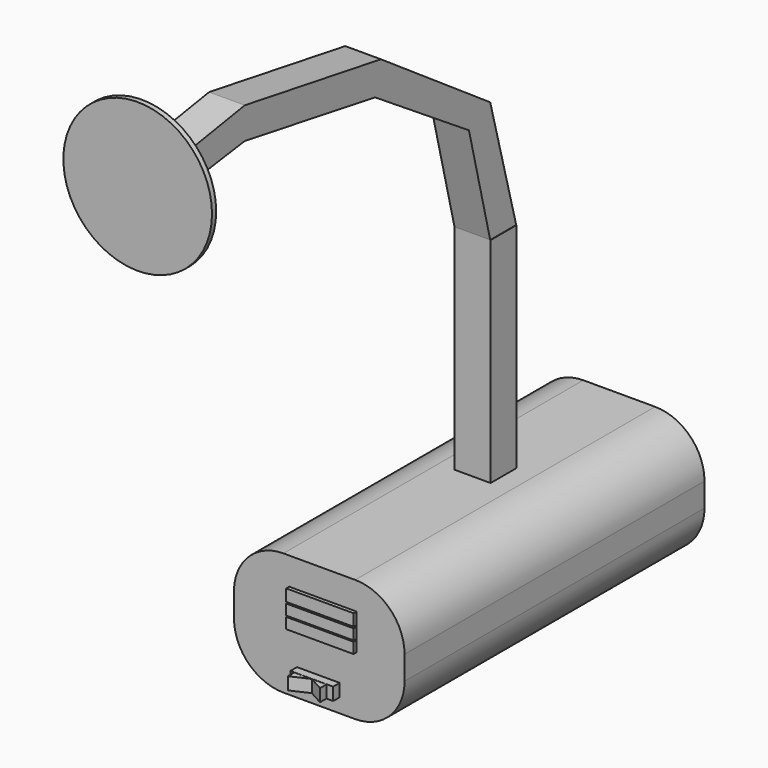
from build123d import *

# Parameters (mm, degrees)
F0_W      = 116.4809949696
F0_H      = 83.6853701621
F1_DEPTH  = 256.032
F2_W      = 24.6532578021
F2_H      = 22.1879333258
F3_DEPTH  = 146.05
F5_DEPTH  = 24.384
F6_R      = 33.7265634664
F9_R      = 50.7557548826
F10_DEPTH = 3.556
F11_W     = 29.1482340544
F11_H     = 8.6365044117
F12_DEPTH = 5.588
F14_DEPTH = 8.5344
F15_W     = 46.036280226
F15_H     = 24.5366059244
F16_DEPTH = 0.762
F17_W     = 46.036280226
F17_H     = 8.0885775387
F18_DEPTH = 1.778
F19_W     = 46.036280226
F19_H     = 7.2142649442
F20_DEPTH = 1.778
F21_W     = 46.036280226
F21_H     = 7.3891170323
F22_DEPTH = 1.778


# Not quite as in the source:
# - the program builds the solid bodies; features that only make, move or delete a surface that nothing else refers to are left out


with BuildPart() as f1:
    # F0 (on Front) → F1 (new body)
    with BuildSketch(Plane.XZ):
        with Locations((23.220455274, -23.1154998764)):
            Rectangle(F0_W, F0_H)
    extrude(amount=-F1_DEPTH)

    # F2 (on face) → F3 (join)
    with BuildSketch(Plane.XY.offset(18.7271852046)):
        with Locations((21.9421936199, 143.5368284583)):
            Rectangle(F2_W, F2_H)
    extrude(amount=F3_DEPTH)

    # F4 (on face) → F5 (join)
    with BuildSketch(Plane(origin=(9.6155647188, 0, 0), x_dir=(0, -1, 0), z_dir=(-1, 0, 0))):
        Polygon((-132.4428617954, 247.5340366364), (-154.6307951212, 164.7771852046), (-132.4428617954, 164.7771852046), (-114.2979115248, 238.0615323782), (-34.0974070132, 290.4760241508), (77.0465955138, 309.4210326672), (149.6690958738, 299.3170320988), (149.6690958738, 318.8935518265), (77.0465955138, 330.8920264244), (-39.1494072974, 311.315536499), align=None)
    extrude(amount=-F5_DEPTH)

    # F6
    f6_edges = [f1.edges().sort_by_distance(p)[0] for p in [
        (-35.020042, 128.016, 18.727185),
        (81.460953, 128.016, 18.727185),
        (-35.020042, 128.016, -64.958185),
        (81.460953, 128.016, -64.958185),
    ]]
    fillet(f6_edges, radius=F6_R)

    # F9 (on face) → F10 (join)
    with BuildSketch(Plane.XZ.offset(149.6690958738)):
        with Locations((21.8075647188, 309.1052919626)):
            Circle(F9_R)
    extrude(amount=F10_DEPTH)

    # F11 (on face) → F12 (join)
    with BuildSketch(Plane.XZ):
        with Locations((22.6024175063, -50.9459078312)):
            Rectangle(F11_W, F11_H)
    extrude(amount=F12_DEPTH)

    # F13 (on face) → F14 (join)
    with BuildSketch(Plane(origin=(0, 0, -55.264160037), x_dir=(1, 0, 0), z_dir=(0, 0, -1))):
        Polygon((32.6312892139, 11.0850147903), (22.6024175063, 5.588), (32.6312892139, 5.588), align=None)
        Polygon((10.6680989265, 11.0850147903), (10.6680989265, 5.588), (22.6024175063, 5.588), align=None)
    extrude(amount=-F14_DEPTH)

    # F15 (on face) → F16 (join)
    with BuildSketch(Plane.XZ):
        with Locations((25.6846474949, -12.2683029622)):
            Rectangle(F15_W, F15_H)
    extrude(amount=F16_DEPTH)

    # F17 (on face) → F18 (join)
    with BuildSketch(Plane.XZ.offset(0.762)):
        with Locations((25.6846474949, -4.0442887694)):
            Rectangle(F17_W, F17_H)
    extrude(amount=F18_DEPTH)

    # F19 (on face) → F20 (join)
    with BuildSketch(Plane.XZ.offset(0.762)):
        with Locations((25.6846474949, -12.7054592595)):
            Rectangle(F19_W, F19_H)
    extrude(amount=F20_DEPTH)

    # F21 (on face) → F22 (join)
    with BuildSketch(Plane.XZ.offset(0.762)):
        with Locations((25.6846474949, -20.8420474082)):
            Rectangle(F21_W, F21_H)
    extrude(amount=F22_DEPTH)


solid = f1.part
